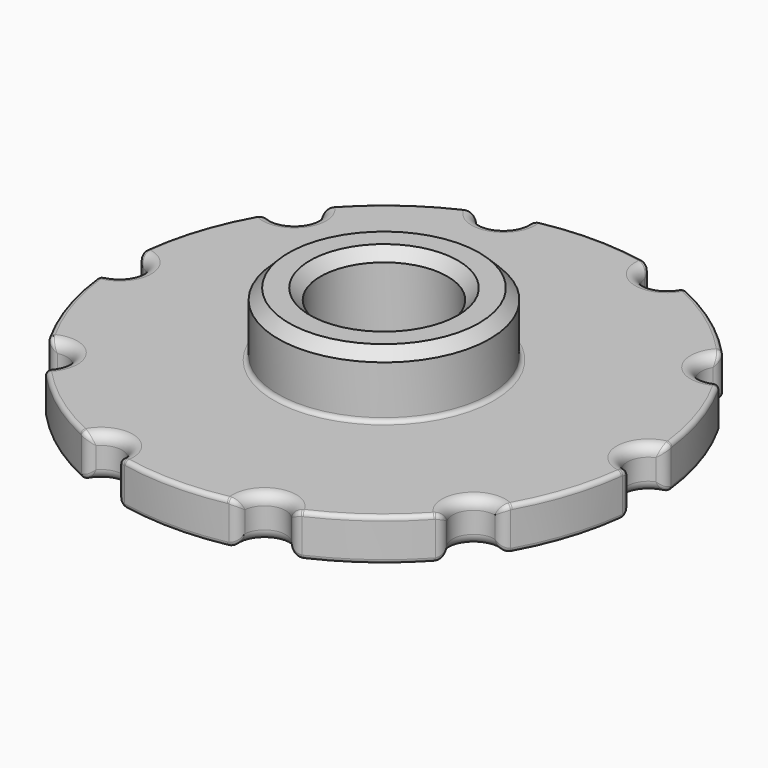
from build123d import *

# Parameters (mm, degrees)
F0_R          = 12.5
F2_DEPTH      = 2
F1_R          = 1
F3_DEPTH      = 2.001
F4_R          = 5
F5_DEPTH      = 3
F6_R          = 3
F7_DEPTH      = 2.001
F7_DEPTH_BACK = 3.001
F8_SIZE       = 0.5
F9_R          = 0.5
F10_R         = 0.2


with BuildPart() as f2:
    # F0 (on Top) → F2 (new body)
    with BuildSketch(Plane.XY):
        Circle(F0_R)
    extrude(amount=F2_DEPTH)

    # F1 (on Top) → F3 (cut, through all)
    with BuildSketch(Plane.XY):
        with Locations((12.5, 0)):
            Circle(F1_R)
        with Locations((10.1127124297, 7.3473156537)):
            Circle(F1_R)
        with Locations((3.8627124297, 11.8882064537)):
            Circle(F1_R)
        with Locations((-3.8627124297, 11.8882064537)):
            Circle(F1_R)
        with Locations((-10.1127124297, 7.3473156537)):
            Circle(F1_R)
        with Locations((-12.5, 0)):
            Circle(F1_R)
        with Locations((-10.1127124297, -7.3473156537)):
            Circle(F1_R)
        with Locations((-3.8627124297, -11.8882064537)):
            Circle(F1_R)
        with Locations((3.8627124297, -11.8882064537)):
            Circle(F1_R)
        with Locations((10.1127124297, -7.3473156537)):
            Circle(F1_R)
    extrude(amount=F3_DEPTH, mode=Mode.SUBTRACT)

    # F4 (on face) → F5 (join)
    with BuildSketch(Plane.XY.offset(2)):
        Circle(F4_R)
    extrude(amount=F5_DEPTH)

    # F6 (on face) → F7 (cut, two sides)
    with BuildSketch(Plane.XY.offset(2)) as f7_sk:
        Circle(F6_R)
    extrude(amount=-F7_DEPTH, mode=Mode.SUBTRACT)
    extrude(f7_sk.sketch, amount=F7_DEPTH_BACK, mode=Mode.SUBTRACT)

    # F8
    f8_edges = [f2.edges().sort_by_distance(p)[0] for p in [
        (-3, 0, 5),
        (-3, 0, 0),
        (-5, 0, 5),
    ]]
    chamfer(f8_edges, length=F8_SIZE)

    # F9
    f9_edges = [f2.edges().sort_by_distance(p)[0] for p in [
        (3.553695, -10.93715, 0),
        (2.900056, -12.158934, 1),
        (3.553695, -10.93715, 2),
        (4.800647, -11.541395, 1),
        (-3.553695, -10.93715, 2),
        (-4.800647, -11.541395, 1),
        (-3.553695, -10.93715, 0),
        (-2.900056, -12.158934, 1),
        (-9.303695, -6.75953, 2),
        (-10.667667, -6.515435, 1),
        (-9.303695, -6.75953, 0),
        (-9.493037, -8.132174, 1),
        (-11.5, 0, 2),
        (-12.46, 0.9992, 1),
        (-11.5, 0, 0),
        (-12.46, -0.9992, 1),
        (-9.303695, 6.75953, 2),
        (-9.493037, 8.132174, 1),
        (-9.303695, 6.75953, 0),
        (-10.667667, 6.515435, 1),
        (-3.553695, 10.93715, 2),
        (-2.900056, 12.158934, 1),
        (-3.553695, 10.93715, 0),
        (-4.800647, 11.541395, 1),
        (3.553695, 10.93715, 0),
        (4.800647, 11.541395, 1),
        (3.553695, 10.93715, 2),
        (2.900056, 12.158934, 1),
        (9.303695, 6.75953, 0),
        (10.667667, 6.515435, 1),
        (9.303695, 6.75953, 2),
        (9.493037, 8.132174, 1),
        (11.5, 0, 0),
        (12.46, -0.9992, 1),
        (11.5, 0, 2),
        (12.46, 0.9992, 1),
        (9.303695, -6.75953, 0),
        (9.493037, -8.132174, 1),
        (9.303695, -6.75953, 2),
        (10.667667, -6.515435, 1),
    ]]
    fillet(f9_edges, radius=F9_R)

    # F10
    f10_edges = [f2.edges().sort_by_distance(p)[0] for p in [
        (11.888206, 3.862712, 0),
        (11, 0, 0),
        (8.899187, 6.465638, 0),
        (11.888206, -3.862712, 0),
        (7.347316, 10.112712, 0),
        (8.899187, -6.465638, 0),
        (3.399187, 10.461622, 0),
        (7.347316, -10.112712, 0),
        (0, 12.5, 0),
        (3.399187, -10.461622, 0),
        (-3.399187, 10.461622, 0),
        (0, -12.5, 0),
        (-7.347316, 10.112712, 0),
        (-3.399187, -10.461622, 0),
        (-8.899187, 6.465638, 0),
        (-7.347316, -10.112712, 0),
        (-11.888206, 3.862712, 0),
        (-8.899187, -6.465638, 0),
        (-11, 0, 0),
        (-11.888206, -3.862712, 0),
        (-3.5, 0, 0),
        (11.888206, -3.862712, 2),
        (8.899187, -6.465638, 2),
        (11, 0, 2),
        (7.347316, -10.112712, 2),
        (11.888206, 3.862712, 2),
        (3.399187, -10.461622, 2),
        (8.899187, 6.465638, 2),
        (0, -12.5, 2),
        (7.347316, 10.112712, 2),
        (-3.399187, -10.461622, 2),
        (3.399187, 10.461622, 2),
        (-7.347316, -10.112712, 2),
        (0, 12.5, 2),
        (-8.899187, -6.465638, 2),
        (-3.399187, 10.461622, 2),
        (-11.888206, -3.862712, 2),
        (-7.347316, 10.112712, 2),
        (-11, 0, 2),
        (-8.899187, 6.465638, 2),
        (-11.888206, 3.862712, 2),
        (-5, 0, 2),
        (12.413371, 1.469091, 0.000805),
        (10.906138, 6.107876, 0.000805),
        (12.413371, 1.469091, 1.999195),
        (10.906138, 6.107876, 1.999195),
        (12.342943, 1.116647, 0.166313),
        (12.342943, -1.116648, 0.166313),
        (12.413371, -1.469091, 0.000805),
        (9.329302, 8.158386, 0.166313),
        (9.179118, 8.484916, 0.000805),
        (10.642, 6.351613, 0.166313),
        (10.906138, -6.107876, 1.999195),
        (12.413371, -1.469091, 1.999195),
        (10.906138, -6.107876, 0.000805),
        (5.233131, 11.351843, 0.000805),
        (9.179118, 8.484916, 1.999195),
        (5.233131, 11.351843, 1.999195),
        (10.641999, -6.351613, 0.166314),
        (9.329302, -8.158387, 0.166313),
        (9.179118, -8.484916, 0.000805),
        (2.752184, 12.083899, 0.166313),
        (2.438754, 12.259791, 0.000805),
        (4.876174, 11.393773, 0.166313),
        (5.233131, -11.351843, 1.999195),
        (9.179118, -8.484916, 1.999195),
        (5.233131, -11.351843, 0.000805),
        (-2.438754, 12.259791, 0.000805),
        (2.438754, 12.259791, 1.999195),
        (-2.438754, 12.259791, 1.999195),
        (4.876174, -11.393773, 0.166314),
        (2.752184, -12.0839, 0.166313),
        (2.438754, -12.259791, 0.000805),
        (-2.752185, 12.083899, 0.166314),
        (-4.876174, 11.393773, 0.166313),
        (-5.233131, 11.351843, 0.000805),
        (-2.438754, -12.259791, 1.999195),
        (2.438754, -12.259791, 1.999195),
        (-2.438754, -12.259791, 0.000805),
        (-9.179118, 8.484916, 0.000805),
        (-5.233131, 11.351843, 1.999195),
        (-9.179118, 8.484916, 1.999195),
        (-4.876174, -11.393773, 0.166313),
        (-5.233131, -11.351843, 0.000805),
        (-2.752184, -12.0839, 0.166313),
        (-9.329302, 8.158386, 0.166314),
        (-10.642, 6.351613, 0.166313),
        (-10.906138, 6.107876, 0.000805),
        (-9.179118, -8.484916, 1.999195),
        (-5.233131, -11.351843, 1.999195),
        (-9.179118, -8.484916, 0.000805),
        (-12.413371, 1.469091, 0.000805),
        (-10.906138, 6.107876, 1.999195),
        (-12.413371, 1.469091, 1.999195),
        (-10.641999, -6.351613, 0.166313),
        (-10.906138, -6.107876, 0.000805),
        (-9.329302, -8.158387, 0.166313),
        (-12.342943, 1.116647, 0.166314),
        (-12.342943, -1.116648, 0.166313),
        (-12.413371, -1.469091, 0.000805),
        (-12.413371, -1.469091, 1.999195),
        (-10.906138, -6.107876, 1.999195),
        (12.342943, 1.116648, 1.833687),
        (10.641999, 6.351613, 1.833686),
        (12.342943, -1.116647, 1.833687),
        (9.329302, 8.158387, 1.833687),
        (9.329302, -8.158387, 1.833687),
        (10.642, -6.351613, 1.833687),
        (4.876174, 11.393773, 1.833686),
        (2.752184, 12.0839, 1.833687),
        (2.752184, -12.083899, 1.833687),
        (4.876174, -11.393773, 1.833687),
        (-2.752185, 12.083899, 1.833686),
        (-4.876174, 11.393773, 1.833687),
        (-4.876174, -11.393773, 1.833687),
        (-2.752184, -12.0839, 1.833687),
        (-9.329302, 8.158386, 1.833686),
        (-10.642, 6.351613, 1.833687),
        (-10.641999, -6.351613, 1.833687),
        (-9.329302, -8.158387, 1.833687),
        (-12.342943, 1.116647, 1.833686),
        (-12.342943, -1.116648, 1.833687),
    ]]
    fillet(f10_edges, radius=F10_R)


solid = f2.part
